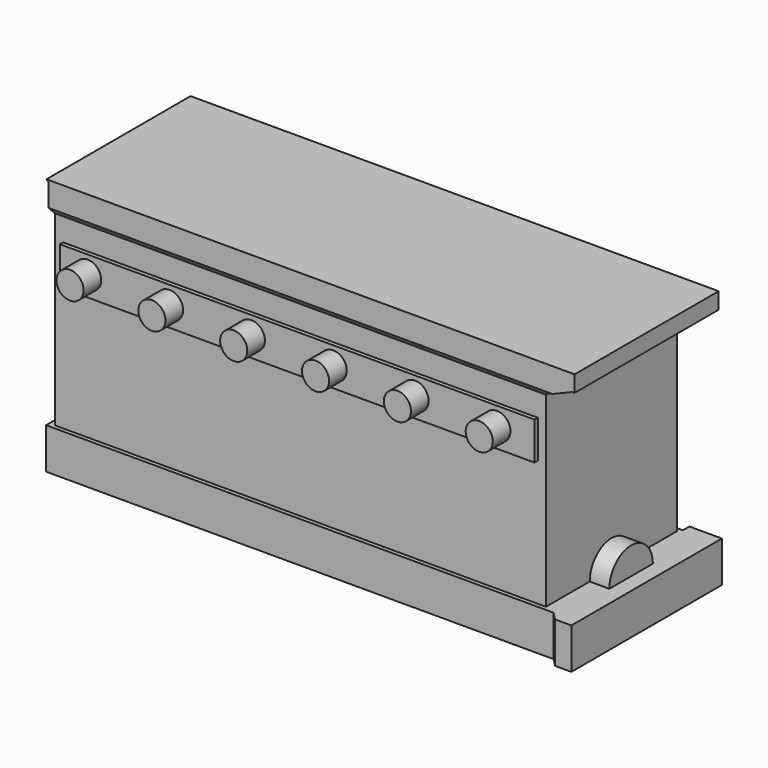
from build123d import *

# Parameters (mm, degrees)
F0_W         = 152.4
F0_H         = 50.8
F0_W_2       = 33.4925577044
F0_H_2       = 31.1666876078
F1_DEPTH     = 63.5
F3_DEPTH     = 26.67
F2_W         = 163.8920905882
F2_H         = 5.08
F4_DEPTH     = 27.94
F2_W_2       = 10.0997969608
F2_H_2       = 12.7
F5_DEPTH     = 29.21
F6_T4_DEPTH  = 152.4
F6_T9_DEPTH  = 152.4
F6_T14_DEPTH = 38.8282991577
F7_T4_DEPTH  = 82.0082991577
F8_SIZE      = 5.08
F9_SIZE      = 5.08
F10_R        = 4.2050090424
F11_DEPTH    = 33.528
F12_W        = 147.32
F12_H        = 11.7464326172
F13_DEPTH    = 26.67
F14_R        = 8.4361197875
F15_DEPTH    = 82.296


# Not quite as in the source:
# - a fillet or chamfer that OpenCascade refuses, or shapes differently, is made with other operations: its cross-section is extruded or revolved along the edge and cut away or added


with BuildPart() as f1:
    # F0 (on Top) → F1 (new body)
    with BuildSketch(Plane.XY):
        Rectangle(F0_W, F0_H)
        with Locations((42.3862338066, 0)):
            Rectangle(F0_W_2, F0_H_2, mode=Mode.SUBTRACT)
    extrude(amount=F1_DEPTH)

    # F2 (on Front) → F3 (join, symmetric)
    with BuildSketch(Plane.XZ):
        Polygon((77.0109159804, 0), (-77.9290840196, 0), (-77.9290840196, -12.7), (4.4760434559, -12.7), (65.76342, -12.7), (77.0109159804, -12.7), align=None)
    extrude(amount=F3_DEPTH, both=True)

    # F2 (on Front) → F4 (join, symmetric)
    with BuildSketch(Plane.XZ):
        with Locations((5.1646676471, 65.5489305882)):
            Rectangle(F2_W, F2_H)
    extrude(amount=F4_DEPTH, both=True)

    # F2 (on Front) → F5 (join, symmetric)
    with BuildSketch(Plane.XZ):
        with Locations((82.0608144608, -6.35)):
            Rectangle(F2_W_2, F2_H_2)
    extrude(amount=F5_DEPTH, both=True)

    # F6: chamfer of 5.08 on 3 edges, made by hand


with BuildPart() as f6_tool2:
    # F6_s3 → F6_t4 (new body)
    with BuildSketch(Plane.YZ.offset(76.2)):
        Polygon((-25.4, 57.9289305882), (-30.48, 63.0089305882), (-25.4, 63.0089305882), align=None)
    extrude(amount=-F6_T4_DEPTH)

    split(bisect_by=Plane.XZ.offset(27.94), keep=Keep.BOTTOM)


with BuildPart() as f1_1:
    add(f1.part)

    # F6_t1: union F6_tool2
    add(f6_tool2.part)


with BuildPart() as f6_tool7:
    # F6_s8 → F6_t9 (new body)
    with BuildSketch(Plane.YZ.offset(-76.2)):
        Polygon((25.4, 57.9289305882), (30.48, 63.0089305882), (25.4, 63.0089305882), align=None)
    extrude(amount=F6_T9_DEPTH)

    split(bisect_by=Plane.XZ.offset(-27.94), keep=Keep.TOP)


with BuildPart() as f1_2:
    add(f1_1.part)

    # F6_t6: union F6_tool7
    add(f6_tool7.part)


with BuildPart() as f6_tool12:
    # F6_s13 → F6_t14 (new body)
    with BuildSketch(Plane.XY.offset(13.0641495789)):
        Polygon((82.0909159804, -29.21), (77.0109159804, -24.13), (77.0109159804, -29.21), align=None)
    extrude(amount=-F6_T14_DEPTH)

    split(bisect_by=Plane.XZ.offset(26.67), keep=Keep.TOP)


with BuildPart() as f1_3:
    add(f1_2.part)

    # F6_t11: cut F6_tool12
    add(f6_tool12.part, mode=Mode.SUBTRACT)

    # F7: chamfer of 5.08 on 1 edges, made by hand


with BuildPart() as f7_tool2:
    # F7_s3 → F7_t4 (new body)
    with BuildSketch(Plane.XZ.offset(-41.0041495789)):
        Polygon((-71.7013776471, 63.0089305882), (-76.7813776471, 68.0889305882), (-76.7813776471, 63.0089305882), align=None)
    extrude(amount=F7_T4_DEPTH)

    split(bisect_by=Plane.YZ.offset(-76.2), keep=Keep.BOTTOM)


with BuildPart() as f1_4:
    add(f1_3.part)

    # F7_t1: cut F7_tool2
    add(f7_tool2.part, mode=Mode.SUBTRACT)

    # F8
    f8_edges = [f1_4.edges().sort_by_distance(p)[0] for p in [
        (76.2, 0, 63.008931),
    ]]
    chamfer(f8_edges, length=F8_SIZE)

    # F9
    f9_edges = [f1_4.edges().sort_by_distance(p)[0] for p in [
        (81.28, 0, 63.008931),
    ]]
    chamfer(f9_edges, length=F9_SIZE)

    # F10 (on Front) → F11 (join)
    with BuildSketch(Plane.XZ):
        with Locations((-65.0145885289, 45.2289305882)):
            Circle(F10_R)
        with Locations((-39.6145885289, 45.2289305882)):
            Circle(F10_R)
        with Locations((-14.2145885289, 45.2289305882)):
            Circle(F10_R)
        with Locations((11.1854114711, 45.2289305882)):
            Circle(F10_R)
        with Locations((36.5854114711, 45.2289305882)):
            Circle(F10_R)
        with Locations((61.9854114711, 45.2289305882)):
            Circle(F10_R)
    extrude(amount=F11_DEPTH)

    # F12 (on Front) → F13 (join)
    with BuildSketch(Plane.XZ):
        with Locations((0, 44.957723322)):
            Rectangle(F12_W, F12_H)
    extrude(amount=F13_DEPTH)

    # F14 (on Right) → F15 (join)
    with BuildSketch(Plane.YZ):
        Circle(F14_R)
    extrude(amount=F15_DEPTH)


solid = f1_4.part
